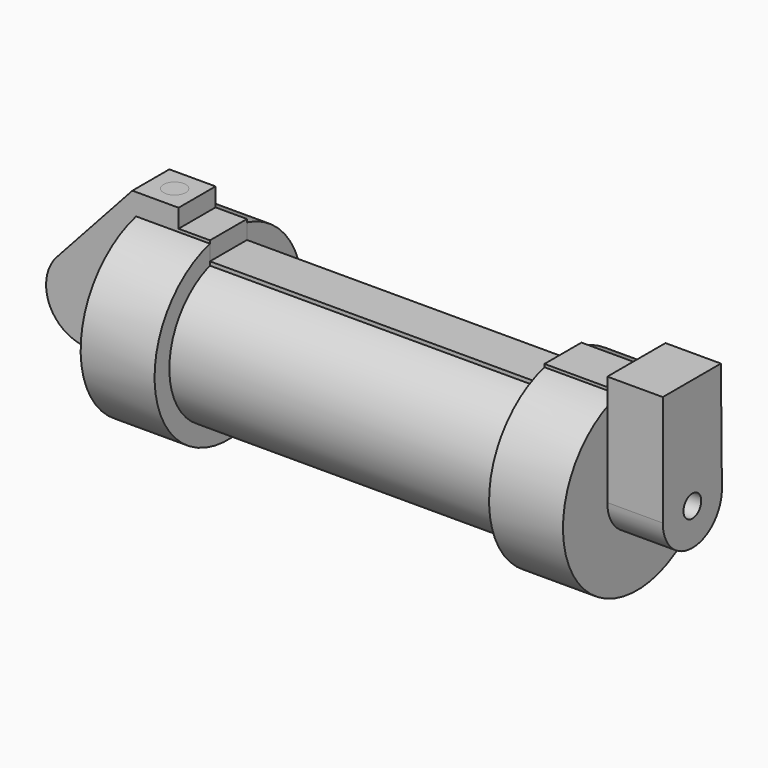
from build123d import *

# Parameters (mm, degrees)
F0_W     = 5.842
F0_H     = 12.7
F0_R     = 3.175
F2_DEPTH = 3.175
F3_R     = 1.524
F4_DEPTH = 7.62
F6_R     = 1.524984407
F7_DEPTH = 17.78
F5_R     = 1.524
F8_DEPTH = 10.414


with BuildPart() as f1:
    # F0 (on Front) → F1 (revolve)
    with BuildSketch(Plane.XZ):
        Polygon((5.842, 12.7), (5.842, 0), (66.294, 0), (66.294, 12.7), (56.134, 12.7), (56.134, 10.16), (10.16, 10.16), (10.16, 12.7), align=None)
        with Locations((2.921, 6.35)):
            Rectangle(F0_W, F0_H)
    revolve(axis=Axis((33.147, 0, 0), (-1, 0, 0)))


with BuildPart() as f2:
    # F0 (on Front) → F2 (new body, symmetric)
    with BuildSketch(Plane.XZ):
        Polygon((5.842, 12.7), (5.842, 0), (66.294, 0), (66.294, 12.7), (56.134, 12.7), (56.134, 10.16), (10.16, 10.16), (10.16, 12.7), align=None)
        with BuildLine():
            ThreePointArc((-8.1826630726, -5.5069827884), (-3.1957909266, -4.5493385486), (-0.9398, 0))
            ThreePointArc((-0.9398, 0), (-4.5919612295, 5.3297205562), (-10.8806298187, 3.8475430269))
            ThreePointArc((-10.8806298187, 3.8475430269), (-12.1459778134, -1.5837270034), (-8.1826630726, -5.5069827884))
        make_face()
        with Locations((-6.6548, 0)):
            Circle(F0_R, mode=Mode.SUBTRACT)
        with BuildLine():
            Line((-0.9398, 0), (0, 0))
            Line((0, 0), (0, 12.7))
            Line((0, 12.7), (5.842, 12.7))
            Line((5.842, 12.7), (5.842, 15.24))
            Line((5.842, 15.24), (-0.508, 15.24))
            Line((-0.508, 15.24), (-10.8806298187, 3.8475430269))
            ThreePointArc((-10.8806298187, 3.8475430269), (-4.5919612295, 5.3297205562), (-0.9398, 0))
        make_face()
        with Locations((2.921, 6.35)):
            Rectangle(F0_W, F0_H)
        with BuildLine():
            Line((5.842, 0), (0, 0))
            Line((0, 0), (-0.9398, 0))
            ThreePointArc((-0.9398, 0), (-3.1957909266, -4.5493385486), (-8.1826630726, -5.5069827884))
            Line((-8.1826630726, -5.5069827884), (5.842, -9.398))
            Line((5.842, -9.398), (5.842, 0))
        make_face()
        with Locations((-6.6548, 0)):
            Circle(F0_R)
    extrude(amount=F2_DEPTH, both=True)


with BuildPart() as f4:
    # F3 (on face) → F4 (new body)
    with BuildSketch(Plane.YZ.offset(66.294)):
        with BuildLine():
            Line((-5.08, 11.6397422652), (-5.08, 0))
            ThreePointArc((-5.08, 0), (-0.0582774056, 5.0796657118), (5.0786628913, 0.1165471414))
            Line((5.0786628913, 0.1165471414), (4.9457994608, 11.6973957655))
            ThreePointArc((4.9457994608, 11.6973957655), (-0.0730303205, 12.6997900208), (-5.08, 11.6397422652))
        make_face()
        with BuildLine():
            Line((-5.08, 15.24), (-5.08, 11.6397422652))
            ThreePointArc((-5.08, 11.6397422652), (-0.0730303205, 12.6997900208), (4.9457994608, 11.6973957655))
            Line((4.9457994608, 11.6973957655), (4.9051562776, 15.24))
            Line((4.9051562776, 15.24), (-5.08, 15.24))
        make_face()
        with BuildLine():
            ThreePointArc((5.0786628913, 0.1165471414), (-0.0582774056, 5.0796657118), (-5.08, 0))
            ThreePointArc((-5.08, 0), (0, -5.08), (5.08, 0))
            Line((5.08, 0), (5.0786628913, 0.1165471414))
        make_face()
        Circle(F3_R, mode=Mode.SUBTRACT)
    extrude(amount=F4_DEPTH)

    # F5 (on face) → F8 (join)
    with BuildSketch(Plane.XY.offset(15.24)):
        with Locations((69.7052180767, 0.1330839295)):
            Circle(F5_R)
    extrude(amount=-F8_DEPTH)


with BuildPart() as f7:
    # F6 (on face) → F7 (new body)
    with BuildSketch(Plane.XY.offset(15.24)):
        with Locations((2.7230642736, 0.0437548333)):
            Circle(F6_R)
    extrude(amount=-F7_DEPTH)


solid = Compound([f1.part, f2.part, f4.part, f7.part])
